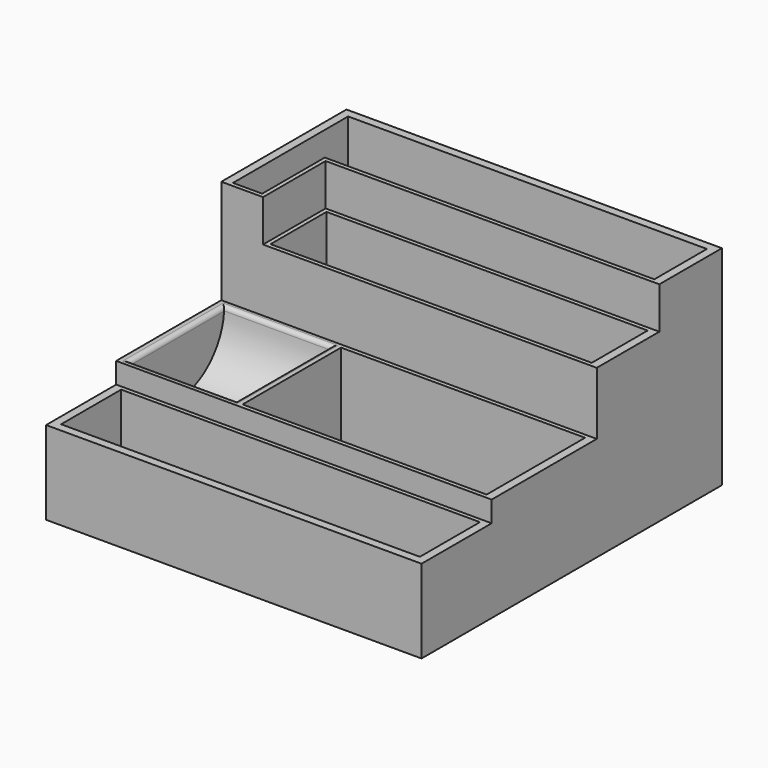
from build123d import *

# Parameters (mm, degrees)
F0_W      = 70
F0_H      = 37.5
F0_W_2    = 90
F1_DEPTH  = 100
F2_DEPTH  = 80
F3_DEPTH  = 50
F0_W_3    = 180
F0_H_2    = 42
F4_DEPTH  = 40
F7_DEPTH  = 55
F8_DEPTH  = 4
F10_R     = 2
F11_W     = 154
F11_H     = 33.5
F11_W_2   = 117
F11_H_2   = 59
F11_W_3   = 172
F11_H_3   = 36
F12_DEPTH = 93


with BuildPart() as f1:
    # F0 (on Top) → F1 (new body)
    with BuildSketch(Plane.XY):
        with Locations((-35, 71.25)):
            Rectangle(F0_W, F0_H)
        with Locations((45, 71.25)):
            Rectangle(F0_W_2, F0_H)
        Polygon((-70, 52.5), (-70, 90), (-90, 90), (-90, 15), (-70, 15), align=None)
    extrude(amount=F1_DEPTH)

    # F0 (on Top) → F2 (join)
    with BuildSketch(Plane.XY):
        with Locations((-35, 33.75)):
            Rectangle(F0_W, F0_H)
        with Locations((45, 33.75)):
            Rectangle(F0_W_2, F0_H)
    extrude(amount=F2_DEPTH)

    # F0 (on Top) → F3 (join)
    with BuildSketch(Plane.XY):
        Polygon((90, -48), (90, 15), (0, 15), (-70, 15), (-90, 15), (-90, -48), align=None)
    extrude(amount=F3_DEPTH)

    # F0 (on Top) → F4 (join)
    with BuildSketch(Plane.XY):
        with Locations((0, -69)):
            Rectangle(F0_W_3, F0_H_2)
    extrude(amount=F4_DEPTH)

    # F6 (on face) → F7 (cut)
    with BuildSketch(Plane(origin=(-90, 0, 0), x_dir=(0, -1, 0), z_dir=(-1, 0, 0))):
        with BuildLine():
            ThreePointArc((-11.75, 50), (16.5, 21.75), (44.75, 50))
            Line((44.75, 50), (-11.75, 50))
        make_face()
    extrude(amount=-F7_DEPTH, mode=Mode.SUBTRACT)

    # F6 (on face) → F8 (join)
    with BuildSketch(Plane(origin=(-90, 0, 0), x_dir=(0, -1, 0), z_dir=(-1, 0, 0))):
        with BuildLine():
            ThreePointArc((-11.75, 50), (16.5, 21.75), (44.75, 50))
            Line((44.75, 50), (-11.75, 50))
        make_face()
    extrude(amount=-F8_DEPTH)

    # F10
    f10_edges = [f1.edges().sort_by_distance(p)[0] for p in [
        (-60.5, 11.75, 50),
        (-35, -16.5, 50),
        (-60.5, -44.75, 50),
        (-86, -16.5, 50),
    ]]
    fillet(f10_edges, radius=F10_R)

    # F11 (on offset) → F12 (cut)
    with BuildSketch(Plane.XY.offset(100)):
        Polygon((-86, 17), (-72, 17), (-72, 52.5), (-72, 54.5), (-70, 54.5), (86, 54.5), (86, 86), (-86, 86), align=None)
        with Locations((9, 33.75)):
            Rectangle(F11_W, F11_H)
        with Locations((27.5, -16.5)):
            Rectangle(F11_W_2, F11_H_2)
        with Locations((0, -68)):
            Rectangle(F11_W_3, F11_H_3)
    extrude(amount=-F12_DEPTH, mode=Mode.SUBTRACT)


solid = f1.part
